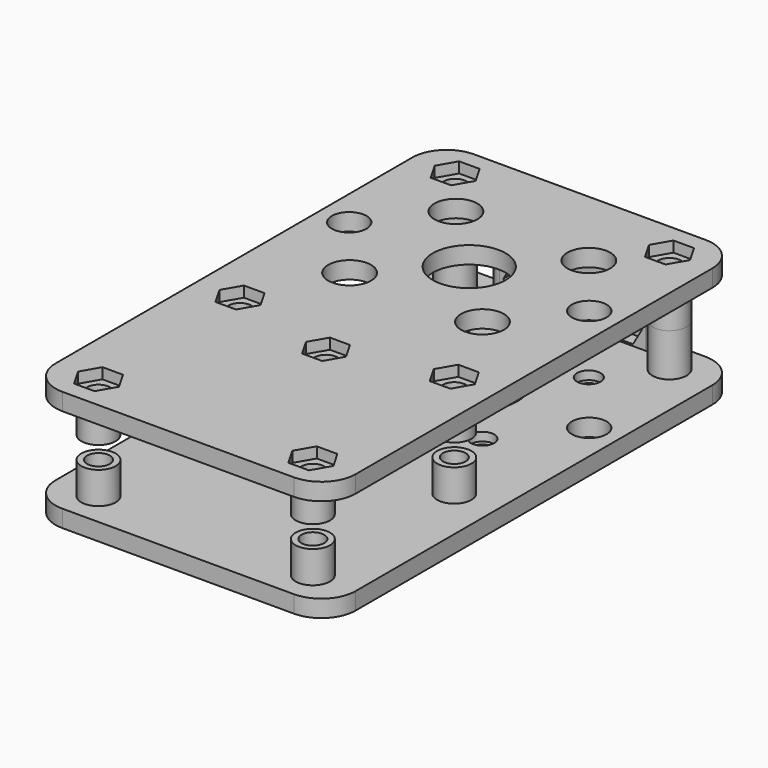
from build123d import *

# Parameters (mm, degrees)
F0_W      = 70
F0_H      = 120
F0_R      = 4.3
F0_R_2    = 4.05
F0_R_3    = 1.65
F0_R_4    = 11.25
F0_R_5    = 2.65
F1_DEPTH  = 4
F2_R      = 2.75
F2_R_2    = 1.65
F3_DEPTH  = 2
F4_DEPTH  = 2.5
F5_DEPTH  = 2.5
F6_R      = 4
F6_R_2    = 2.65
F7_DEPTH  = 7.45
F8_DEPTH  = 10
F10_DEPTH = 10
F11_R     = 2.15
F12_DEPTH = 5
F13_R     = 2.15
F14_DEPTH = 3
F16_DEPTH = 2.5
F17_R     = 5
F17_R_2   = 1.65
F18_DEPTH = 4
F17_R_3   = 11.25
F17_R_4   = 8.5
F19_DEPTH = 4
F20_R     = 2.65
F21_DEPTH = 2.5
F22_DEPTH = 2.5
F23_R     = 2.65
F24_DEPTH = 2.5
F25_R     = 8
F25_2_R   = 8


# Not quite as in the source:
# - a feature names something its author has since deleted; it is built from what else it names


with BuildPart() as f1:
    # F0 (on Top) → F1 (new body)
    with BuildSketch(Plane.XY):
        Rectangle(F0_W, F0_H)
        with Locations((-25, -52)):
            Circle(F0_R, mode=Mode.SUBTRACT)
        with Locations((-25, -10.75)):
            Circle(F0_R, mode=Mode.SUBTRACT)
        with Locations((25, -52)):
            Circle(F0_R, mode=Mode.SUBTRACT)
        with Locations((0, -16.9)):
            Circle(F0_R, mode=Mode.SUBTRACT)
        with Locations((25, -10.75)):
            Circle(F0_R, mode=Mode.SUBTRACT)
        with Locations((-28, 24.85)):
            Circle(F0_R_2, mode=Mode.SUBTRACT)
        with Locations((-15.5, 9.35)):
            Circle(F0_R_3, mode=Mode.SUBTRACT)
        with Locations((-25, 52)):
            Circle(F0_R, mode=Mode.SUBTRACT)
        with Locations((-15.5, 40.35)):
            Circle(F0_R_3, mode=Mode.SUBTRACT)
        with Locations((15.5, 9.35)):
            Circle(F0_R_3, mode=Mode.SUBTRACT)
        with Locations((0, 24.85)):
            Circle(F0_R_4, mode=Mode.SUBTRACT)
        with Locations((28, 24.85)):
            Circle(F0_R_2, mode=Mode.SUBTRACT)
        with Locations((15.5, 40.35)):
            Circle(F0_R_3, mode=Mode.SUBTRACT)
        with Locations((25, 52)):
            Circle(F0_R, mode=Mode.SUBTRACT)
        with Locations((25, 52)):
            Circle(F0_R)
        with Locations((25, 52)):
            Circle(F0_R_5, mode=Mode.SUBTRACT)
        with Locations((-25, 52)):
            Circle(F0_R)
        with Locations((-25, 52)):
            Circle(F0_R_5, mode=Mode.SUBTRACT)
        with Locations((25, -10.75)):
            Circle(F0_R)
        with Locations((25, -10.75)):
            Circle(F0_R_5, mode=Mode.SUBTRACT)
        with Locations((-25, -10.75)):
            Circle(F0_R)
        with Locations((-25, -10.75)):
            Circle(F0_R_5, mode=Mode.SUBTRACT)
        with Locations((25, -52)):
            Circle(F0_R)
        with Locations((25, -52)):
            Circle(F0_R_5, mode=Mode.SUBTRACT)
        with Locations((-25, -52)):
            Circle(F0_R)
        with Locations((-25, -52)):
            Circle(F0_R_5, mode=Mode.SUBTRACT)
        with Locations((0, -16.9)):
            Circle(F0_R)
        with Locations((0, -16.9)):
            Circle(F0_R_5, mode=Mode.SUBTRACT)
    extrude(amount=F1_DEPTH)

    # F2 (on face) → F3 (cut)
    with BuildSketch(Plane.XY.offset(4)):
        with Locations((-15.5, 40.35)):
            Circle(F2_R)
        with Locations((-15.5, 40.35)):
            Circle(F2_R_2, mode=Mode.SUBTRACT)
        with Locations((-15.5, 9.35)):
            Circle(F2_R)
        with Locations((-15.5, 9.35)):
            Circle(F2_R_2, mode=Mode.SUBTRACT)
        with Locations((15.5, 9.35)):
            Circle(F2_R)
        with Locations((15.5, 9.35)):
            Circle(F2_R_2, mode=Mode.SUBTRACT)
        with Locations((15.5, 40.35)):
            Circle(F2_R)
        with Locations((15.5, 40.35)):
            Circle(F2_R_2, mode=Mode.SUBTRACT)
    extrude(amount=-F3_DEPTH, mode=Mode.SUBTRACT)

    # F0 (on Top) → F4 (cut)
    with BuildSketch(Plane.XY):
        with Locations((25, 52)):
            Circle(F0_R)
        with Locations((25, 52)):
            Circle(F0_R_5, mode=Mode.SUBTRACT)
        with Locations((-25, 52)):
            Circle(F0_R)
        with Locations((-25, 52)):
            Circle(F0_R_5, mode=Mode.SUBTRACT)
        with Locations((25, -10.75)):
            Circle(F0_R)
        with Locations((25, -10.75)):
            Circle(F0_R_5, mode=Mode.SUBTRACT)
        with Locations((-25, -10.75)):
            Circle(F0_R)
        with Locations((-25, -10.75)):
            Circle(F0_R_5, mode=Mode.SUBTRACT)
        with Locations((25, -52)):
            Circle(F0_R)
        with Locations((25, -52)):
            Circle(F0_R_5, mode=Mode.SUBTRACT)
        with Locations((-25, -52)):
            Circle(F0_R)
        with Locations((-25, -52)):
            Circle(F0_R_5, mode=Mode.SUBTRACT)
    extrude(amount=F4_DEPTH, mode=Mode.SUBTRACT)

    # F0 (on Top) → F5 (cut)
    with BuildSketch(Plane.XY):
        with Locations((0, -16.9)):
            Circle(F0_R)
        with Locations((0, -16.9)):
            Circle(F0_R_5, mode=Mode.SUBTRACT)
    extrude(amount=F5_DEPTH, mode=Mode.SUBTRACT)

    # F6 (on face) → F7 (join)
    with BuildSketch(Plane.XY.offset(4)):
        with Locations((-25, -10.75)):
            Circle(F6_R)
        with Locations((-25, -10.75)):
            Circle(F6_R_2, mode=Mode.SUBTRACT)
        with Locations((-25, -52)):
            Circle(F6_R)
        with Locations((-25, -52)):
            Circle(F6_R_2, mode=Mode.SUBTRACT)
        with Locations((25, -52)):
            Circle(F6_R)
        with Locations((25, -52)):
            Circle(F6_R_2, mode=Mode.SUBTRACT)
        with Locations((25, -10.75)):
            Circle(F6_R)
        with Locations((25, -10.75)):
            Circle(F6_R_2, mode=Mode.SUBTRACT)
        with Locations((0, -16.9)):
            Circle(F6_R)
        with Locations((0, -16.9)):
            Circle(F6_R_2, mode=Mode.SUBTRACT)
    extrude(amount=F7_DEPTH)

    # F6 (on face) → F8 (join)
    with BuildSketch(Plane.XY.offset(4)):
        with Locations((-25, 52)):
            Circle(F6_R)
        with Locations((-25, 52)):
            Circle(F6_R_2, mode=Mode.SUBTRACT)
        with Locations((25, 52)):
            Circle(F6_R)
        with Locations((25, 52)):
            Circle(F6_R_2, mode=Mode.SUBTRACT)
    extrude(amount=F8_DEPTH)

    # F9 (on face) → F10 (join)
    with BuildSketch(Plane.XY.offset(4)):
        with BuildLine():
            Line((20, 60), (-20, 60))
            Line((-20, 60), (-20, 58))
            ThreePointArc((-20, 58), (-19.1213203436, 55.8786796564), (-17, 55))
            Line((-17, 55), (17, 55))
            ThreePointArc((17, 55), (19.1213203436, 55.8786796564), (20, 58))
            Line((20, 58), (20, 60))
        make_face()
    extrude(amount=F10_DEPTH)

    # F11 (on face) → F12 (cut, through all)
    with BuildSketch(Plane(origin=(0, 60, 0), x_dir=(-1, 0, 0), z_dir=(0, 1, 0))):
        with Locations((12, 8)):
            Circle(F11_R)
        with Locations((-12, 8)):
            Circle(F11_R)
    extrude(amount=-F12_DEPTH, mode=Mode.SUBTRACT)

    # F13 (on face) → F14 (cut)
    with BuildSketch(Plane.XZ.offset(-55)):
        Polygon((14.0784609691, 11.6), (9.9215390309, 11.6), (7.8430780618, 8), (9.9215390309, 4.4), (14.0784609691, 4.4), (16.1569219382, 8), align=None)
        with Locations((12, 8)):
            Circle(F13_R, mode=Mode.SUBTRACT)
        Polygon((-9.9215390309, 11.6), (-14.0784609691, 11.6), (-16.1569219382, 8), (-14.0784609691, 4.4), (-9.9215390309, 4.4), (-7.8430780618, 8), align=None)
        with Locations((-12, 8)):
            Circle(F13_R, mode=Mode.SUBTRACT)
    extrude(amount=-F14_DEPTH, mode=Mode.SUBTRACT)


with BuildPart() as f15_1:
    # F15: instance of F1
    add(f1.part.mirror(Plane(origin=(-25, 52, 14), x_dir=(1, 0, 0), z_dir=(0, 0, 1))))

    # F16 (add, through all): faces of the model
    f16_faces = [f15_1.faces().sort_by_distance(p)[0] for p in [
        (-29.1783776336, -10.75, 25.5),
        (-29.1783776336, -52, 25.5),
        (20.8216223664, -52, 25.5),
        (20.8216223664, -10.75, 25.5),
        (-29.1783776336, 52, 25.5),
        (20.8216223664, 52, 25.5),
    ]]
    extrude(f16_faces, amount=F16_DEPTH)

    # F17 (on face) → F18 (cut, through all)
    with BuildSketch(Plane.XY.offset(28)):
        with Locations((-15.5, 40.35)):
            Circle(F17_R)
        with Locations((-15.5, 40.35)):
            Circle(F17_R_2, mode=Mode.SUBTRACT)
        with Locations((15.5, 40.35)):
            Circle(F17_R)
        with Locations((15.5, 40.35)):
            Circle(F17_R_2, mode=Mode.SUBTRACT)
        with Locations((15.5, 9.35)):
            Circle(F17_R)
        with Locations((15.5, 9.35)):
            Circle(F17_R_2, mode=Mode.SUBTRACT)
        with Locations((-15.5, 9.35)):
            Circle(F17_R)
        with Locations((-15.5, 9.35)):
            Circle(F17_R_2, mode=Mode.SUBTRACT)
    extrude(amount=-F18_DEPTH, mode=Mode.SUBTRACT)

    # F17 (on face) → F19 (join, through all)
    with BuildSketch(Plane.XY.offset(28)):
        with Locations((0, 24.85)):
            Circle(F17_R_3)
        with Locations((0, 24.85)):
            Circle(F17_R_4, mode=Mode.SUBTRACT)
    extrude(amount=-F19_DEPTH)

    # F20 (on face) → F21 (cut)
    with BuildSketch(Plane.XY.offset(28)):
        Polygon((-22.6039963829, 56.15), (-27.3960036171, 56.15), (-29.7920072343, 52), (-27.3960036171, 47.85), (-22.6039963829, 47.85), (-20.2079927657, 52), align=None)
        with Locations((-25, 52)):
            Circle(F20_R, mode=Mode.SUBTRACT)
        Polygon((27.3960036171, 56.15), (22.6039963829, 56.15), (20.2079927657, 52), (22.6039963829, 47.85), (27.3960036171, 47.85), (29.7920072343, 52), align=None)
        with Locations((25, 52)):
            Circle(F20_R, mode=Mode.SUBTRACT)
        Polygon((27.3960036171, -6.6), (22.6039963829, -6.6), (20.2079927657, -10.75), (22.6039963829, -14.9), (27.3960036171, -14.9), (29.7920072343, -10.75), align=None)
        with Locations((25, -10.75)):
            Circle(F20_R, mode=Mode.SUBTRACT)
        Polygon((-22.6039963829, -6.6), (-27.3960036171, -6.6), (-29.7920072343, -10.75), (-27.3960036171, -14.9), (-22.6039963829, -14.9), (-20.2079927657, -10.75), align=None)
        with Locations((-25, -10.75)):
            Circle(F20_R, mode=Mode.SUBTRACT)
        Polygon((-22.6039963829, -47.85), (-27.3960036171, -47.85), (-29.7920072343, -52), (-27.3960036171, -56.15), (-22.6039963829, -56.15), (-20.2079927657, -52), align=None)
        with Locations((-25, -52)):
            Circle(F20_R, mode=Mode.SUBTRACT)
        Polygon((27.3960036171, -47.85), (22.6039963829, -47.85), (20.2079927657, -52), (22.6039963829, -56.15), (27.3960036171, -56.15), (29.7920072343, -52), align=None)
        with Locations((25, -52)):
            Circle(F20_R, mode=Mode.SUBTRACT)
    extrude(amount=-F21_DEPTH, mode=Mode.SUBTRACT)

    # F22 (add, through all): a face of the model
    f22_faces = [f15_1.faces().sort_by_distance(p)[0] for p in [
        (-4.1783776336, -16.9, 25.5),
    ]]
    extrude(f22_faces, amount=F22_DEPTH)

    # F23 (on face) → F24 (cut)
    with BuildSketch(Plane.XY.offset(28)):
        Polygon((2.3382685902, -12.85), (-2.3382685902, -12.85), (-4.6765371804, -16.9), (-2.3382685902, -20.95), (2.3382685902, -20.95), (4.6765371804, -16.9), align=None)
        with Locations((0, -16.9)):
            Circle(F23_R, mode=Mode.SUBTRACT)
    extrude(amount=-F24_DEPTH, mode=Mode.SUBTRACT)

    # F25
    f25_edges = [f15_1.edges().sort_by_distance(p)[0] for p in [
        (-35, 60, 26),
        (35, 60, 26),
        (35, -60, 26),
        (-35, -60, 26),
    ]]
    fillet(f25_edges, radius=F25_R)


with BuildPart() as f1_1:
    add(f1.part)

    # F25#2
    f25_2_edges = [f1_1.edges().sort_by_distance(p)[0] for p in [
        (35, 60, 2),
        (-35, 60, 2),
        (-35, -60, 2),
        (35, -60, 2),
    ]]
    fillet(f25_2_edges, radius=F25_2_R)


solid = Compound([f15_1.part, f1_1.part])
